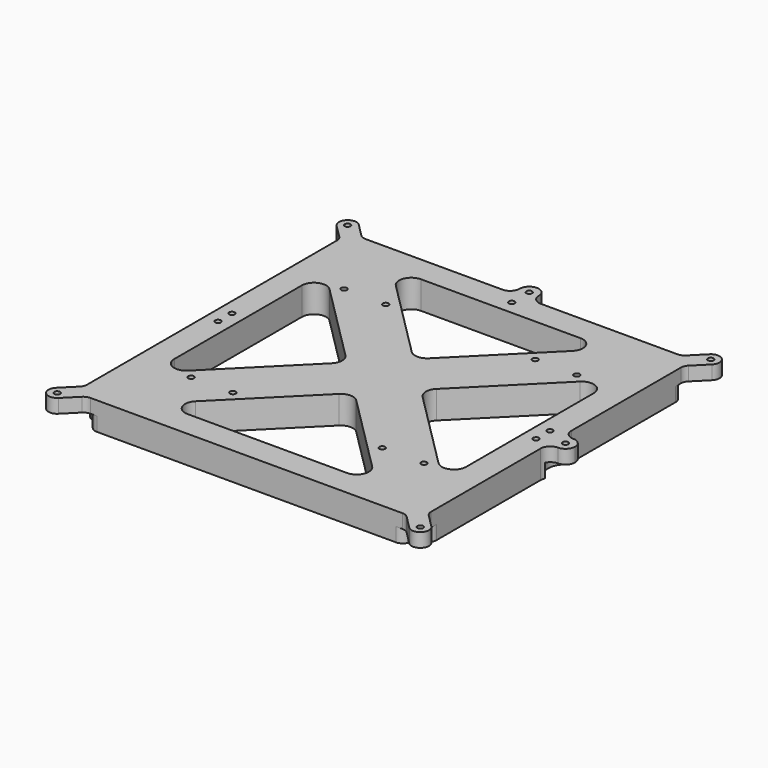
from build123d import *

# Parameters (mm, degrees)
F0_W         = 198
F0_H         = 198
F1_DEPTH     = 16
F2_W         = 11
F2_H         = 11
F3_DEPTH     = 16
F5_DEPTH     = 8
F6_R         = 5
F7_R         = 7
F8_T1_DEPTH  = 35.5
F8_T3_DEPTH  = 8
F8_T8_DEPTH  = 35.5
F8_S11_R     = 10
F8_T12_DEPTH = 20
F8_T16_DEPTH = 35.5
F8_S19_R     = 10
F8_T20_DEPTH = 20
F8_T24_DEPTH = 35.5
F8_S27_R     = 10
F8_T28_DEPTH = 20
F8_T32_DEPTH = 35.5
F8_S35_R     = 10
F8_T36_DEPTH = 20
F9_D         = 3.3
F10_D        = 3.3
F11_D        = 3.3


# Not quite as in the source:
# - a fillet or chamfer that OpenCascade refuses, or shapes differently, is made with other operations: its cross-section is extruded or revolved along the edge and cut away or added
# - ends of sketch curves that miss each other by under 0.0002 mm in the source are joined
# - a feature names something its author has since deleted; it is built from what else it names


with BuildPart() as f1:
    # F0 (on Top) → F1 (new body)
    with BuildSketch(Plane.XY):
        Rectangle(F0_W, F0_H)
        Polygon((-62.7867965644, -84), (0, -21.2132034356), (62.7867965644, -84), align=None, mode=Mode.SUBTRACT)
        Polygon((84, -62.7867965644), (21.2132034356, 0), (84, 62.7867965644), align=None, mode=Mode.SUBTRACT)
        Polygon((-84, 62.7867965644), (-21.2132034356, 0), (-84, -62.7867965644), align=None, mode=Mode.SUBTRACT)
        Polygon((62.7867965644, 84), (0, 21.2132034356), (-62.7867965644, 84), align=None, mode=Mode.SUBTRACT)
    extrude(amount=F1_DEPTH)

    # F2 (on face) → F3 (join, through all)
    with BuildSketch(Plane.XY.offset(16)):
        with BuildLine():
            Line((-99, -99), (-99, -91.9289296269))
            Line((-99, -91.9289296269), (-108.0355351865, -100.9644648135))
            ThreePointArc((-108.0355351865, -100.9644648135), (-108.0355351865, -108.0355351865), (-100.9644648135, -108.0355351865))
            Line((-100.9644648135, -108.0355351865), (-91.9289321881, -99))
            Line((-91.9289321881, -99), (-99, -99))
        make_face()
        with BuildLine():
            Line((99, -99), (91.9289321881, -99))
            Line((91.9289321881, -99), (100.9644660941, -108.0355339059))
            ThreePointArc((100.9644660941, -108.0355339059), (108.0355351865, -108.0355351865), (108.0355351865, -100.9644648135))
            Line((108.0355351865, -100.9644648135), (99, -91.9289296269))
            Line((99, -91.9289296269), (99, -99))
        make_face()
        with Locations((104.5, 0)):
            Rectangle(F2_W, F2_H)
        with BuildLine():
            Line((100.9644660941, 108.0355339059), (91.9289321881, 99))
            Line((91.9289321881, 99), (99, 99))
            Line((99, 99), (99, 91.9289296269))
            Line((99, 91.9289296269), (108.0355351865, 100.9644648135))
            ThreePointArc((108.0355351865, 100.9644648135), (108.0355351865, 108.0355351865), (100.9644660941, 108.0355339059))
        make_face()
        with BuildLine():
            Line((-99, 99), (-91.9289321881, 99))
            Line((-91.9289321881, 99), (-100.9644660941, 108.0355339059))
            ThreePointArc((-100.9644660941, 108.0355339059), (-108.0355351865, 108.0355351865), (-108.0355351865, 100.9644648135))
            Line((-108.0355351865, 100.9644648135), (-99, 91.9289296269))
            Line((-99, 91.9289296269), (-99, 99))
        make_face()
        with Locations((0, 104.5)):
            Rectangle(F2_W, F2_H)
    extrude(amount=-F3_DEPTH)

    # F4 (on face) → F5 (cut)
    with BuildSketch(Plane(origin=(0, 0, 0), x_dir=(1, 0, 0), z_dir=(0, 0, -1))):
        with BuildLine():
            Line((-99, 91.9289296269), (-99, 89.5562516017))
            ThreePointArc((-99, 89.5562516017), (-92.9111652352, 92.9111652352), (-89.5562516017, 99))
            Line((-89.5562516017, 99), (-91.9289321881, 99))
            Line((-91.9289321881, 99), (-100.9644648135, 108.0355351865))
            ThreePointArc((-100.9644648135, 108.0355351865), (-108.0355351865, 108.0355351865), (-108.0355351865, 100.9644648135))
            Line((-108.0355351865, 100.9644648135), (-99, 91.9289296269))
        make_face()
        with BuildLine():
            Line((91.9289321881, 99), (89.5562516017, 99))
            ThreePointArc((89.5562516017, 99), (92.9111652352, 92.9111652352), (99, 89.5562516017))
            Line((99, 89.5562516017), (99, 91.9289296269))
            Line((99, 91.9289296269), (108.0355351865, 100.9644648135))
            ThreePointArc((108.0355351865, 100.9644648135), (108.0355358268, 108.0355345462), (100.9644660941, 108.0355339059))
            Line((100.9644660941, 108.0355339059), (91.9289321881, 99))
        make_face()
        with BuildLine():
            ThreePointArc((-89.5562516017, -99), (-92.9111652352, -92.9111652352), (-99, -89.5562516017))
            Line((-99, -89.5562516017), (-99, -91.9289296269))
            Line((-99, -91.9289296269), (-108.0355351865, -100.9644648135))
            ThreePointArc((-108.0355351865, -100.9644648135), (-108.0355358268, -108.0355345462), (-100.9644660941, -108.0355339059))
            Line((-100.9644660941, -108.0355339059), (-91.9289321881, -99))
            Line((-91.9289321881, -99), (-89.5562516017, -99))
        make_face()
        with BuildLine():
            Line((99, 5.5), (99, 8.3516465442))
            ThreePointArc((99, 8.3516465442), (94.5, 0), (99, -8.3516465442))
            Line((99, -8.3516465442), (99, -5.5))
            Line((99, -5.5), (110, -5.5))
            Line((110, -5.5), (110, 5.5))
            Line((110, 5.5), (99, 5.5))
        make_face()
        with BuildLine():
            ThreePointArc((114.5, 0), (109.2434164903, 8.8034084308), (99, 8.3516465442))
            Line((99, 8.3516465442), (99, 5.5))
            Line((99, 5.5), (110, 5.5))
            Line((110, 5.5), (110, -5.5))
            Line((110, -5.5), (99, -5.5))
            Line((99, -5.5), (99, -8.3516465442))
            ThreePointArc((99, -8.3516465442), (109.2434164903, -8.8034084308), (114.5, 0))
        make_face()
        with BuildLine():
            Line((-5.5, -99), (-8.3516465442, -99))
            ThreePointArc((-8.3516465442, -99), (-2.8708478327, -114.0790517652), (10, -104.5))
            ThreePointArc((10, -104.5), (9.5790517652, -101.6291521673), (8.3516465442, -99))
            Line((8.3516465442, -99), (5.5, -99))
            Line((5.5, -99), (5.5, -110))
            Line((5.5, -110), (-5.5, -110))
            Line((-5.5, -110), (-5.5, -99))
        make_face()
        with BuildLine():
            ThreePointArc((8.3516465442, -99), (0, -94.5), (-8.3516465442, -99))
            Line((-8.3516465442, -99), (-5.5, -99))
            Line((-5.5, -99), (-5.5, -110))
            Line((-5.5, -110), (5.5, -110))
            Line((5.5, -110), (5.5, -99))
            Line((5.5, -99), (8.3516465442, -99))
        make_face()
        with BuildLine():
            Line((99, -91.9289296269), (99, -89.5562516017))
            ThreePointArc((99, -89.5562516017), (92.9111652352, -92.9111652352), (89.5562516017, -99))
            Line((89.5562516017, -99), (91.9289321881, -99))
            Line((91.9289321881, -99), (100.9644660941, -108.0355339059))
            ThreePointArc((100.9644660941, -108.0355339059), (108.0355358268, -108.0355345462), (108.0355351865, -100.9644648135))
            Line((108.0355351865, -100.9644648135), (99, -91.9289296269))
        make_face()
    extrude(amount=-F5_DEPTH, mode=Mode.SUBTRACT)

    # F6
    f6_edges = [f1.edges().sort_by_distance(p)[0] for p in [
        (-91.928932, 99, 12),
        (-99, 91.92893, 12),
        (-99, -91.92893, 12),
        (-91.928932, -99, 12),
        (91.928932, -99, 12),
        (99, -91.92893, 12),
        (99, 91.92893, 12),
        (91.928932, 99, 12),
        (89.556252, 99, 4),
        (99, 89.556252, 4),
        (99, -89.556252, 4),
        (89.556252, -99, 4),
        (-89.556252, -99, 4),
        (-99, -89.556252, 4),
        (-89.556252, 99, 4),
        (-99, 89.556252, 4),
    ]]
    fillet(f6_edges, radius=F6_R)

    # F7
    f7_edges = [f1.edges().sort_by_distance(p)[0] for p in [
        (-84, -62.786797, 8),
        (-84, 62.786797, 8),
        (-21.213203, 0, 8),
        (62.786797, -84, 8),
        (-62.786797, -84, 8),
        (0, -21.213203, 8),
        (21.213203, 0, 8),
        (84, -62.786797, 8),
        (84, 62.786797, 8),
        (62.786797, 84, 8),
        (0, 21.213203, 8),
        (-62.786797, 84, 8),
    ]]
    fillet(f7_edges, radius=F7_R)

    # F8: fillet of radius 5.5 on 8 edges, made by hand

    # F8_s2 → F8_t1 (cut)
    with BuildSketch(Plane.XY.offset(-5.75)):
        with BuildLine():
            ThreePointArc((104.5, -5.5), (108.3890872965, -3.8890872965), (110, 0))
            Line((110, 0), (110, -5.5))
            Line((110, -5.5), (104.5, -5.5))
        make_face()
        with BuildLine():
            ThreePointArc((104.5, 5.5), (108.3890872965, 3.8890872965), (110, 0))
            Line((110, 0), (110, 5.5))
            Line((110, 5.5), (104.5, 5.5))
        make_face()
        with BuildLine():
            ThreePointArc((-5.5, 104.5), (-3.8890872965, 108.3890872965), (0, 110))
            Line((0, 110), (-5.5, 110))
            Line((-5.5, 110), (-5.5, 104.5))
        make_face()
        with BuildLine():
            ThreePointArc((5.5, 104.5), (3.8890872965, 108.3890872965), (0, 110))
            Line((0, 110), (5.5, 110))
            Line((5.5, 110), (5.5, 104.5))
        make_face()
    extrude(amount=F8_T1_DEPTH, mode=Mode.SUBTRACT)

    # F8_s4 → F8_t3 (join)
    with BuildSketch(Plane.XY.offset(8)):
        with BuildLine():
            ThreePointArc((104.5, -5.5), (100.6109127035, -7.1109127035), (99, -11))
            Line((99, -11), (99, -5.5))
            Line((99, -5.5), (104.5, -5.5))
        make_face()
        with BuildLine():
            ThreePointArc((104.5, 5.5), (100.6109127035, 7.1109127035), (99, 11))
            Line((99, 11), (99, 5.5))
            Line((99, 5.5), (104.5, 5.5))
        make_face()
        with BuildLine():
            ThreePointArc((-5.5, 104.5), (-7.1109127035, 100.6109127035), (-11, 99))
            Line((-11, 99), (-5.5, 99))
            Line((-5.5, 99), (-5.5, 104.5))
        make_face()
        with BuildLine():
            ThreePointArc((5.5, 104.5), (7.1109127035, 100.6109127035), (11, 99))
            Line((11, 99), (5.5, 99))
            Line((5.5, 99), (5.5, 104.5))
        make_face()
    extrude(amount=F8_T3_DEPTH)


with BuildPart() as f8_tool6:
    # F8_s7 → F8_t8 (new body)
    with BuildSketch(Plane.XY.offset(29.75)):
        with BuildLine():
            ThreePointArc((104.5, -5.5), (100.6109127035, -7.1109127035), (99, -11))
            Line((99, -11), (99, -5.5))
            Line((99, -5.5), (104.5, -5.5))
        make_face()
    extrude(amount=-F8_T8_DEPTH)

    split(bisect_by=Plane.XY, keep=Keep.TOP)

    split(bisect_by=Plane.XY.offset(8), keep=Keep.BOTTOM)

    # F8_s11 → F8_t12 (cut, symmetric)
    with BuildSketch(Plane.XY.offset(12)):
        with Locations((104.5, 0)):
            Circle(F8_S11_R)
    extrude(amount=F8_T12_DEPTH, both=True, mode=Mode.SUBTRACT)


with BuildPart() as f1_1:
    add(f1.part)

    # F8_t5: union F8_tool6
    add(f8_tool6.part)


with BuildPart() as f8_tool14:
    # F8_s15 → F8_t16 (new body)
    with BuildSketch(Plane.XY.offset(29.75)):
        with BuildLine():
            ThreePointArc((104.5, 5.5), (100.6109127035, 7.1109127035), (99, 11))
            Line((99, 11), (99, 5.5))
            Line((99, 5.5), (104.5, 5.5))
        make_face()
    extrude(amount=-F8_T16_DEPTH)

    split(bisect_by=Plane.XY, keep=Keep.TOP)

    split(bisect_by=Plane.XY.offset(8), keep=Keep.BOTTOM)

    # F8_s19 → F8_t20 (cut, symmetric)
    with BuildSketch(Plane.XY.offset(12)):
        with Locations((104.5, 0)):
            Circle(F8_S19_R)
    extrude(amount=F8_T20_DEPTH, both=True, mode=Mode.SUBTRACT)


with BuildPart() as f1_2:
    add(f1_1.part)

    # F8_t13: union F8_tool14
    add(f8_tool14.part)


with BuildPart() as f8_tool22:
    # F8_s23 → F8_t24 (new body)
    with BuildSketch(Plane.XY.offset(29.75)):
        with BuildLine():
            ThreePointArc((-5.5, 104.5), (-7.1109127035, 100.6109127035), (-11, 99))
            Line((-11, 99), (-5.5, 99))
            Line((-5.5, 99), (-5.5, 104.5))
        make_face()
    extrude(amount=-F8_T24_DEPTH)

    split(bisect_by=Plane.XY, keep=Keep.TOP)

    split(bisect_by=Plane.XY.offset(8), keep=Keep.BOTTOM)

    # F8_s27 → F8_t28 (cut, symmetric)
    with BuildSketch(Plane.XY.offset(12)):
        with Locations((0, 104.5)):
            Circle(F8_S27_R)
    extrude(amount=F8_T28_DEPTH, both=True, mode=Mode.SUBTRACT)


with BuildPart() as f1_3:
    add(f1_2.part)

    # F8_t21: union F8_tool22
    add(f8_tool22.part)


with BuildPart() as f8_tool30:
    # F8_s31 → F8_t32 (new body)
    with BuildSketch(Plane.XY.offset(29.75)):
        with BuildLine():
            ThreePointArc((5.5, 104.5), (7.1109127035, 100.6109127035), (11, 99))
            Line((11, 99), (5.5, 99))
            Line((5.5, 99), (5.5, 104.5))
        make_face()
    extrude(amount=-F8_T32_DEPTH)

    split(bisect_by=Plane.XY, keep=Keep.TOP)

    split(bisect_by=Plane.XY.offset(8), keep=Keep.BOTTOM)

    # F8_s35 → F8_t36 (cut, symmetric)
    with BuildSketch(Plane.XY.offset(12)):
        with Locations((0, 104.5)):
            Circle(F8_S35_R)
    extrude(amount=F8_T36_DEPTH, both=True, mode=Mode.SUBTRACT)


with BuildPart() as f1_4:
    add(f1_3.part)

    # F8_t29: union F8_tool30
    add(f8_tool30.part)

    # F9 (through all)
    with Locations(Plane.XY.offset(16)):
        with Locations((104.5, 104.5), (-104.5, 104.5), (-104.5, -104.5), (104.5, -104.5), (0, 104.5), (104.5, 0), (91.5, -5), (91.5, 5), (-91.5, -5), (-91.5, 5)):
            Hole(F9_D / 2)

    # F10 (through all)
    with Locations(Plane(origin=(0, 0, 0), x_dir=(1, 0, 0), z_dir=(0, 0, -1))):
        with Locations((67, 55), (43, 55), (-43, 55), (-67, 55), (-67, -55), (-43, -55), (43, -55), (67, -55)):
            Hole(F10_D / 2)

    # F11 (through all)
    with Locations(Plane(origin=(0, 0, 0), x_dir=(1, 0, 0), z_dir=(0, 0, -1))):
        with Locations((0, -91.9289290905)):
            Hole(F11_D / 2)


solid = f1_4.part
